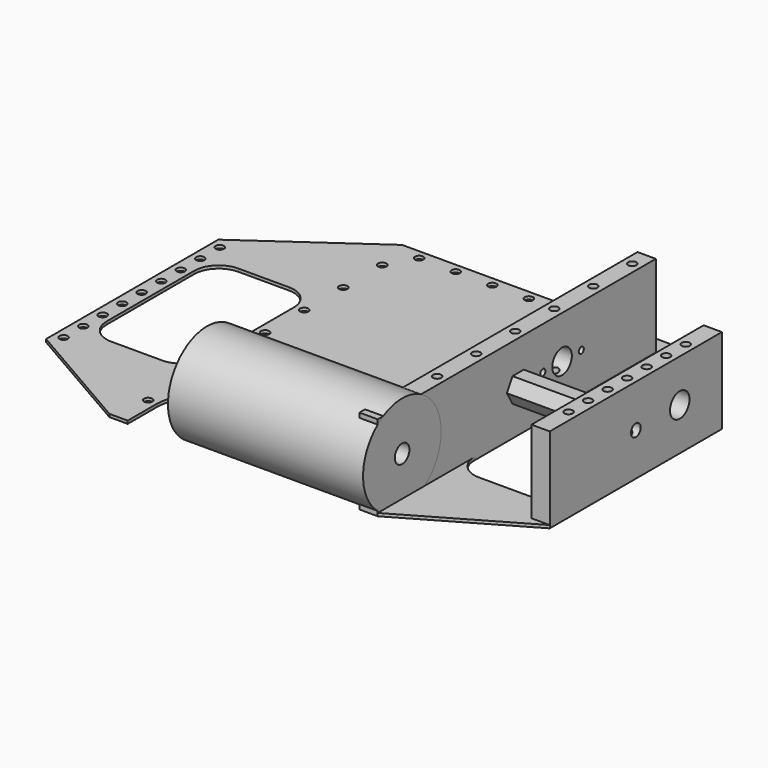
from build123d import *

# Parameters (mm, degrees)
F3_DEPTH  = 1.524
F4_D      = 4.318
F5_W      = 51.7495162792
F5_H      = 82.55
F6_DEPTH  = 1.524
F7_R      = 12.7
F8_R      = 19.05
F9_W      = 9.525
F9_H      = 180.975
F9_R      = 2.159
F10_DEPTH = 44.45
F9_H_2    = 112.0462830635
F11_R     = 3.175
F11_R_2   = 6.35
F12_DEPTH = 70.7995162792
F13_R     = 4.7625
F14_DEPTH = 51.7495162792
F16_D     = 3.3
F17_R     = 4.7625
F17_R_2   = 3.175
F18_DEPTH = 51.7495162792
F19_R     = 25.4
F19_R_2   = 4.7625
F20_DEPTH = 101.6
F21_D     = 10.0838


with BuildPart() as f3:
    # F1 (on Top) → F3 (new body)
    with BuildSketch(Plane.XY):
        Polygon((131.1245162792, 56.0231415318), (69.85, 99.1), (0, 99.1), (-69.85, 99.1), (-131.1245162792, 56.0231415318), (-131.1245162792, -56.0231415318), (-69.85, -91.4), (-60.325, -91.4), (-60.325, -53.3), (0, -53.3), (60.325, -53.3), (60.325, -91.4), (69.85, -91.4), (131.1245162792, -56.0231415318), align=None)
    extrude(amount=F3_DEPTH)

    # F4 (through all)
    with Locations(Plane(origin=(0, 0, 0), x_dir=(1, 0, 0), z_dir=(0, 0, -1))):
        with Locations((19.05, -94.3375), (38.1, -94.3375), (57.15, -94.3375), (65.0875, -80.2382752299), (65.0875, -54.8382752299), (65.0875, -29.4382752299), (65.0875, -4.0382752299), (65.0875, 21.3617247701), (65.0875, 46.7617247701), (65.0875, 72.1617247701), (126.3620162792, 37.8238802177), (126.3620162792, 25.1238802177), (126.3620162792, 12.4238802177), (126.3620162792, -0.2761197823), (126.3620162792, -12.9761197823), (126.3620162792, -25.6761197823), (126.3620162792, -38.3761197823), (-126.3620162792, -25.6761197823), (-126.3620162792, 12.4238802177), (-126.3620162792, 25.1238802177), (-126.3620162792, 50.5238802177), (-126.3620162792, 37.8238802177), (-126.3620162792, -38.3761197823), (-126.3620162792, -0.2761197823), (-126.3620162792, -51.0761197823), (-126.3620162792, -12.9761197823), (-38.1, -94.3375), (-57.15, -94.3375), (-19.05, -94.3375), (-65.0875, -80.2382752299), (-65.0875, -29.4382752299), (-65.0875, 46.7617247701), (-65.0875, -4.0382752299), (-65.0875, -54.8382752299), (-65.0875, 72.1617247701), (-65.0875, 21.3617247701), (0, -94.3375)):
            Hole(F4_D / 2)

    # F5 (on Top) → F6 (cut, through all)
    with BuildSketch(Plane.XY):
        with Locations((95.7247581396, 0)):
            Rectangle(F5_W, F5_H)
        with Locations((-95.7247581396, 0)):
            Rectangle(F5_W, F5_H)
    extrude(amount=F6_DEPTH, mode=Mode.SUBTRACT)

    # F7
    f7_edges = [f3.edges().sort_by_distance(p)[0] for p in [
        (-69.85, 41.275, 0.762),
        (-121.599516, 41.275, 0.762),
        (69.85, -41.275, 0.762),
        (-121.599516, -41.275, 0.762),
        (121.599516, -41.275, 0.762),
        (-69.85, -41.275, 0.762),
        (121.599516, 41.275, 0.762),
        (69.85, 41.275, 0.762),
    ]]
    fillet(f7_edges, radius=F7_R)

    # F8
    f8_edges = [f3.edges().sort_by_distance(p)[0] for p in [
        (-60.325, -53.3, 0.762),
        (60.325, -53.3, 0.762),
    ]]
    fillet(f8_edges, radius=F8_R)


with BuildPart() as f10:
    # F9 (on Top) → F10 (new body)
    with BuildSketch(Plane.XY):
        with Locations((65.0875, -0.9125)):
            Rectangle(F9_W, F9_H)
        with Locations((65.0875, -72.1617247701)):
            Circle(F9_R, mode=Mode.SUBTRACT)
        with Locations((65.0875, -46.7617247701)):
            Circle(F9_R, mode=Mode.SUBTRACT)
        with Locations((65.0875, -21.3617247701)):
            Circle(F9_R, mode=Mode.SUBTRACT)
        with Locations((65.0875, 4.0382752299)):
            Circle(F9_R, mode=Mode.SUBTRACT)
        with Locations((65.0875, 29.4382752299)):
            Circle(F9_R, mode=Mode.SUBTRACT)
        with Locations((65.0875, 54.8382752299)):
            Circle(F9_R, mode=Mode.SUBTRACT)
        with Locations((65.0875, 80.2382752299)):
            Circle(F9_R, mode=Mode.SUBTRACT)
    extrude(amount=F10_DEPTH)


with BuildPart() as f10b:
    # F9 (on Top) → F10, piece 2 (new body)
    with BuildSketch(Plane.XY):
        with Locations((126.3620162792, 0)):
            Rectangle(F9_W, F9_H_2)
        with Locations((126.3620162792, -37.8238802177)):
            Circle(F9_R, mode=Mode.SUBTRACT)
        with Locations((126.3620162792, -25.1238802177)):
            Circle(F9_R, mode=Mode.SUBTRACT)
        with Locations((126.3620162792, -12.4238802177)):
            Circle(F9_R, mode=Mode.SUBTRACT)
        with Locations((126.3620162792, 0.2761197823)):
            Circle(F9_R, mode=Mode.SUBTRACT)
        with Locations((126.3620162792, 12.9761197823)):
            Circle(F9_R, mode=Mode.SUBTRACT)
        with Locations((126.3620162792, 25.6761197823)):
            Circle(F9_R, mode=Mode.SUBTRACT)
        with Locations((126.3620162792, 38.3761197823)):
            Circle(F9_R, mode=Mode.SUBTRACT)
    extrude(amount=F10_DEPTH)


with BuildPart() as f12_tool:
    # F11 (on face) → F12 (new body, through all)
    with BuildSketch(Plane.YZ.offset(131.1245162792)):
        with Locations((0, 22.225)):
            Circle(F11_R)
        with Locations((28.575, 22.225)):
            Circle(F11_R_2)
    extrude(amount=-F12_DEPTH)


with BuildPart() as f10_1:
    add(f10.part)

    # F12: cut by f12_tool
    add(f12_tool.part, mode=Mode.SUBTRACT)

    # F16 (through all)
    with Locations(Plane(origin=(60.325, 0, 0), x_dir=(0, -1, 0), z_dir=(-1, 0, 0))):
        with Locations((-16.075, 22.225), (-41.075, 22.225)):
            Hole(F16_D / 2)

    # F21 (through all)
    with Locations(Plane.YZ.offset(69.85)):
        with Locations((-75.525, 22.225)):
            Hole(F21_D / 2)


with BuildPart() as f10b_1:
    add(f10b.part)

    # F12: cut by f12_tool
    add(f12_tool.part, mode=Mode.SUBTRACT)


with BuildPart() as f14:
    # F13 (on face) → F14 (new body, through all)
    with BuildSketch(Plane.YZ.offset(69.85)):
        Polygon((7.3323484187, 22.225), (3.6661742094, 28.575), (-3.6661742094, 28.575), (-7.3323484187, 22.225), (-3.6661742094, 15.875), (3.6661742094, 15.875), align=None)
        with Locations((0, 22.225)):
            Circle(F13_R, mode=Mode.SUBTRACT)
    extrude(amount=F14_DEPTH)


with BuildPart() as f18:
    # F17 (on face) → F18 (new body, through all)
    with BuildSketch(Plane.YZ.offset(69.85)):
        with Locations((0, 22.225)):
            Circle(F17_R)
        with Locations((0, 22.225)):
            Circle(F17_R_2, mode=Mode.SUBTRACT)
    extrude(amount=F18_DEPTH)


with BuildPart() as f20:
    # F19 (on face) → F20 (new body)
    with BuildSketch(Plane.YZ.offset(69.85)):
        with Locations((-75.525, 22.225)):
            Circle(F19_R)
        with Locations((-75.525, 22.225)):
            Circle(F19_R_2, mode=Mode.SUBTRACT)
    extrude(amount=-F20_DEPTH)


solid = Compound([f3.part, f10_1.part, f10b_1.part, f14.part, f18.part, f20.part])
